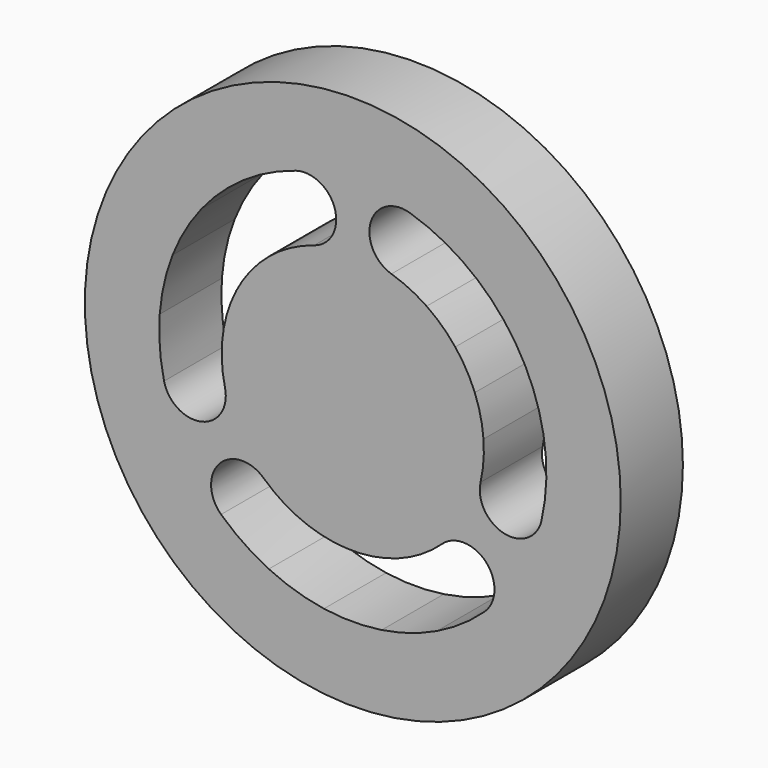
from build123d import *

# Parameters (mm, degrees)
F0_R     = 38.1
F1_DEPTH = 11.049
F3_DEPTH = 11.05


with BuildPart() as f1:
    # F0 (on Front) → F1 (new body)
    with BuildSketch(Plane.XZ):
        Circle(F0_R)
    extrude(amount=F1_DEPTH)

    # F2 (on face) → F3 (cut, through all)
    with BuildSketch(Plane.XZ.offset(11.049)):
        with BuildLine():
            ThreePointArc((-5.4934258743, 17.8092492746), (-3.2271754935, 19.4172396715), (-2.3586126245, 22.0567703964))
            ThreePointArc((-2.3586126245, 22.0567703964), (-4.1640818997, 25.6332075274), (-8.1137993748, 26.3042915181))
            ThreePointArc((-8.1137993748, 26.3042915181), (-10.0430162679, 25.1004998579), (-11.1244292478, 23.1001153577))
            ThreePointArc((-11.1244292478, 23.1001153577), (-9.253900361, 21.4598737334), (-8.5576944102, 19.0714499485))
            ThreePointArc((-8.5576944102, 19.0714499485), (-8.5888494373, 18.5460952541), (-8.681877787, 18.0281049871))
            ThreePointArc((-8.681877787, 18.0281049871), (-7.108001728, 17.6222047723), (-5.4934258743, 17.8092492746))
        make_face()
        with BuildLine():
            ThreePointArc((-11.1244292478, 23.1001153577), (-10.0430162679, 25.1004998579), (-8.1137993748, 26.3042915181))
            ThreePointArc((-8.1137993748, 26.3042915181), (-11.9436262917, 24.8011952044), (-15.5066523142, 22.7440811326))
            ThreePointArc((-15.5066523142, 22.7440811326), (-13.36264294, 23.5018519681), (-11.1244292478, 23.1001153577))
        make_face()
        with BuildLine():
            ThreePointArc((-10.498736832, 15.3988185422), (-8.0863997604, 16.7915820124), (-5.4934258743, 17.8092492746))
            ThreePointArc((-5.4934258743, 17.8092492746), (-7.108001728, 17.6222047723), (-8.681877787, 18.0281049871))
            ThreePointArc((-8.681877787, 18.0281049871), (-9.34582792, 16.5445244505), (-10.498736832, 15.3988185422))
        make_face()
        with BuildLine():
            ThreePointArc((-8.5576944102, 19.0714499485), (-9.253900361, 21.4598737334), (-11.1244292478, 23.1001153577))
            ThreePointArc((-11.1244292478, 23.1001153577), (-10.8084192424, 20.128157176), (-8.681877787, 18.0281049871))
            ThreePointArc((-8.681877787, 18.0281049871), (-8.5888494373, 18.5460952541), (-8.5576944102, 19.0714499485))
        make_face()
        with BuildLine():
            ThreePointArc((-8.681877787, 18.0281049871), (-10.8084192424, 20.128157176), (-11.1244292478, 23.1001153577))
            ThreePointArc((-11.1244292478, 23.1001153577), (-13.36264294, 23.5018519681), (-15.5066523142, 22.7440811326))
            ThreePointArc((-15.5066523142, 22.7440811326), (-16.9953355125, 21.0251239305), (-17.4390806002, 18.7948589632))
            ThreePointArc((-17.4390806002, 18.7948589632), (-14.7880141659, 17.4149152983), (-13.6100435462, 14.6681384642))
            ThreePointArc((-13.6100435462, 14.6681384642), (-11.986449243, 14.7441793583), (-10.498736832, 15.3988185422))
            ThreePointArc((-10.498736832, 15.3988185422), (-9.34582792, 16.5445244505), (-8.681877787, 18.0281049871))
        make_face()
        with BuildLine():
            ThreePointArc((-17.4390806002, 18.7948589632), (-16.9953355125, 21.0251239305), (-15.5066523142, 22.7440811326))
            ThreePointArc((-15.5066523142, 22.7440811326), (-18.7232851045, 20.178902038), (-21.5216706751, 17.1629596491))
            ThreePointArc((-21.5216706751, 17.1629596491), (-19.696270544, 18.5190225314), (-17.4390806002, 18.7948589632))
        make_face()
        with BuildLine():
            ThreePointArc((-14.571188844, 11.6201352503), (-12.6765494203, 13.6620709396), (-10.498736832, 15.3988185422))
            ThreePointArc((-10.498736832, 15.3988185422), (-11.986449243, 14.7441793583), (-13.6100435462, 14.6681384642))
            ThreePointArc((-13.6100435462, 14.6681384642), (-13.6035837106, 14.5299100198), (-13.6014297362, 14.391547479))
            ThreePointArc((-13.6014297362, 14.391547479), (-13.8508683455, 12.9234570127), (-14.571188844, 11.6201352503))
        make_face()
        with BuildLine():
            ThreePointArc((-13.6100435462, 14.6681384642), (-14.7880141659, 17.4149152983), (-17.4390806002, 18.7948589632))
            ThreePointArc((-17.4390806002, 18.7948589632), (-16.2611099805, 16.0480821291), (-13.6100435462, 14.6681384642))
        make_face()
        with BuildLine():
            ThreePointArc((-13.6100435462, 14.6681384642), (-16.2611099805, 16.0480821291), (-17.4390806002, 18.7948589632))
            ThreePointArc((-17.4390806002, 18.7948589632), (-19.696270544, 18.5190225314), (-21.5216706751, 17.1629596491))
            ThreePointArc((-21.5216706751, 17.1629596491), (-22.437544489, 15.0815737307), (-22.2041931112, 12.8195968699))
            ThreePointArc((-22.2041931112, 12.8195968699), (-19.2641605846, 12.2823757795), (-17.3288972096, 10.0048434687))
            ThreePointArc((-17.3288972096, 10.0048434687), (-15.7998480839, 10.5560689065), (-14.571188844, 11.6201352503))
            ThreePointArc((-14.571188844, 11.6201352503), (-13.8508683455, 12.9234570127), (-13.6014297362, 14.391547479))
            ThreePointArc((-13.6014297362, 14.391547479), (-13.6035837106, 14.5299100198), (-13.6100435462, 14.6681384642))
        make_face()
        with BuildLine():
            ThreePointArc((-22.2041931112, 12.8195968699), (-22.437544489, 15.0815737307), (-21.5216706751, 17.1629596491))
            ThreePointArc((-21.5216706751, 17.1629596491), (-23.8392977721, 13.7636250419), (-25.6243943624, 10.0568338021))
            ThreePointArc((-25.6243943624, 10.0568338021), (-24.2797981866, 11.8906966911), (-22.2041931112, 12.8195968699))
        make_face()
        with BuildLine():
            ThreePointArc((-17.3489268741, 6.8089517461), (-16.1403320456, 9.3186248461), (-14.571188844, 11.6201352503))
            ThreePointArc((-14.571188844, 11.6201352503), (-15.7998480839, 10.5560689065), (-17.3288972096, 10.0048434687))
            ThreePointArc((-17.3288972096, 10.0048434687), (-17.114059345, 9.2318818452), (-17.0416605846, 8.4328928597))
            ThreePointArc((-17.0416605846, 8.4328928597), (-17.1191526371, 7.6065156285), (-17.3489268741, 6.8089517461))
        make_face()
        with BuildLine():
            ThreePointArc((-17.3288972096, 10.0048434687), (-19.2641605846, 12.2823757795), (-22.2041931112, 12.8195968699))
            ThreePointArc((-22.2041931112, 12.8195968699), (-20.2689297362, 10.5420645591), (-17.3288972096, 10.0048434687))
        make_face()
        with BuildLine():
            ThreePointArc((-17.3288972096, 10.0048434687), (-20.2689297362, 10.5420645591), (-22.2041931112, 12.8195968699))
            ThreePointArc((-22.2041931112, 12.8195968699), (-24.2797981866, 11.8906966911), (-25.6243943624, 10.0568338021))
            ThreePointArc((-25.6243943624, 10.0568338021), (-25.8860792444, 7.7979594331), (-24.9963656228, 5.7052573369))
            ThreePointArc((-24.9963656228, 5.7052573369), (-22.028601796, 6.0584932723), (-19.5080023094, 4.4525742255))
            ThreePointArc((-19.5080023094, 4.4525742255), (-18.209361165, 5.4300053303), (-17.3489268741, 6.8089517461))
            ThreePointArc((-17.3489268741, 6.8089517461), (-17.1191526371, 7.6065156285), (-17.0416605846, 8.4328928597))
            ThreePointArc((-17.0416605846, 8.4328928597), (-17.114059345, 9.2318818452), (-17.3288972096, 10.0048434687))
        make_face()
        with BuildLine():
            ThreePointArc((-24.9963656228, 5.7052573369), (-25.8860792444, 7.7979594331), (-25.6243943624, 10.0568338021))
            ThreePointArc((-25.6243943624, 10.0568338021), (-26.8370843559, 6.1253894436), (-27.4502782232, 2.0571140049))
            ThreePointArc((-27.4502782232, 2.0571140049), (-26.7059592707, 4.205830226), (-24.9963656228, 5.7052573369))
        make_face()
        with BuildLine():
            ThreePointArc((-18.5851364875, 1.3927631904), (-18.1699752899, 4.1471780197), (-17.3489268741, 6.8089517461))
            ThreePointArc((-17.3489268741, 6.8089517461), (-18.209361165, 5.4300053303), (-19.5080023094, 4.4525742255))
            ThreePointArc((-19.5080023094, 4.4525742255), (-18.81302758, 3.1667060392), (-18.5727073475, 1.7249387027))
            ThreePointArc((-18.5727073475, 1.7249387027), (-18.5758157193, 1.5587347207), (-18.5851364875, 1.3927631904))
        make_face()
        with BuildLine():
            ThreePointArc((-19.5080023094, 4.4525742255), (-22.028601796, 6.0584932723), (-24.9963656228, 5.7052573369))
            ThreePointArc((-24.9963656228, 5.7052573369), (-22.4757661361, 4.09933829), (-19.5080023094, 4.4525742255))
        make_face()
        with BuildLine():
            ThreePointArc((-19.5080023094, 4.4525742255), (-22.4757661361, 4.09933829), (-24.9963656228, 5.7052573369))
            ThreePointArc((-24.9963656228, 5.7052573369), (-26.7059592707, 4.205830226), (-27.4502782232, 2.0571140049))
            ThreePointArc((-27.4502782232, 2.0571140049), (-27.0345222544, -0.1785378544), (-25.567501354, -1.9160193477))
            ThreePointArc((-25.567501354, -1.9160193477), (-22.835705067, -0.7037129493), (-19.9537357944, -1.4953257775))
            ThreePointArc((-19.9537357944, -1.4953257775), (-19.0008925012, -0.1785379824), (-18.5851364875, 1.3927631904))
            ThreePointArc((-18.5851364875, 1.3927631904), (-18.5758157193, 1.5587347207), (-18.5727073475, 1.7249387027))
            ThreePointArc((-18.5727073475, 1.7249387027), (-18.81302758, 3.1667060392), (-19.5080023094, 4.4525742255))
        make_face()
        with BuildLine():
            ThreePointArc((-25.567501354, -1.9160193477), (-27.0345222544, -0.1785378544), (-27.4502782232, 2.0571140049))
            ThreePointArc((-27.4502782232, 2.0571140049), (-27.4502782273, -2.0571139506), (-26.8370843706, -6.1253893792))
            ThreePointArc((-26.8370843706, -6.1253893792), (-26.7591786586, -3.8527427103), (-25.567501354, -1.9160193477))
        make_face()
        with BuildLine():
            ThreePointArc((-18.1699752313, -4.1471782764), (-18.5851364598, -1.3927635598), (-18.5851364875, 1.3927631904))
            ThreePointArc((-18.5851364875, 1.3927631904), (-19.0008925012, -0.1785379824), (-19.9537357944, -1.4953257775))
            ThreePointArc((-19.9537357944, -1.4953257775), (-18.8152778676, -2.6553923195), (-18.1699752313, -4.1471782764))
        make_face()
        with BuildLine():
            ThreePointArc((-19.9537357944, -1.4953257775), (-22.835705067, -0.7037129493), (-25.567501354, -1.9160193477))
            ThreePointArc((-25.567501354, -1.9160193477), (-22.6855320815, -2.7076321758), (-19.9537357944, -1.4953257775))
        make_face()
        with BuildLine():
            ThreePointArc((-19.9537357944, -1.4953257775), (-22.6855320815, -2.7076321758), (-25.567501354, -1.9160193477))
            ThreePointArc((-25.567501354, -1.9160193477), (-26.7591786586, -3.8527427103), (-26.8370843706, -6.1253893792))
            ThreePointArc((-26.8370843706, -6.1253893792), (-22.0058477047, -9.5533346008), (-18.058529801, -5.1362838278))
            ThreePointArc((-18.058529801, -5.1362838278), (-18.086479028, -4.6386017315), (-18.1699752313, -4.1471782764))
            ThreePointArc((-18.1699752313, -4.1471782764), (-18.8152778676, -2.6553923195), (-19.9537357944, -1.4953257775))
        make_face()
        with BuildLine():
            ThreePointArc((-11.2718580074, -16.5327792097), (-11.7072761395, -14.9668124528), (-12.676549357, -13.6620709983))
            ThreePointArc((-12.676549357, -13.6620709983), (-18.9583327467, -13.8971187492), (-18.7232849958, -20.1789021388))
            ThreePointArc((-18.7232849958, -20.1789021388), (-16.7161623907, -21.2477571476), (-14.4430721062, -21.18409601))
            ThreePointArc((-14.4430721062, -21.18409601), (-13.6876442891, -18.292430993), (-11.2718580074, -16.5327792097))
        make_face()
        with BuildLine():
            ThreePointArc((-8.0863997947, -16.7915819959), (-10.4987367878, -15.3988185723), (-12.676549357, -13.6620709983))
            ThreePointArc((-12.676549357, -13.6620709983), (-11.7072761395, -14.9668124528), (-11.2718580074, -16.5327792097))
            ThreePointArc((-11.2718580074, -16.5327792097), (-9.6550645989, -16.3659866159), (-8.0863997947, -16.7915819959))
        make_face()
        with BuildLine():
            ThreePointArc((-14.4430721062, -21.18409601), (-16.7161623907, -21.2477571476), (-18.7232849958, -20.1789021388))
            ThreePointArc((-18.7232849958, -20.1789021388), (-15.5066520681, -22.7440813004), (-11.9436261572, -24.8011952692))
            ThreePointArc((-11.9436261572, -24.8011952692), (-13.6718794549, -23.3233141096), (-14.4430721062, -21.18409601))
        make_face()
        with BuildLine():
            ThreePointArc((-8.0863997947, -16.7915819959), (-9.6550645989, -16.3659866159), (-11.2718580074, -16.5327792097))
            ThreePointArc((-11.2718580074, -16.5327792097), (-11.2591544038, -16.7264479204), (-11.2549171764, -16.9204865685))
            ThreePointArc((-11.2549171764, -16.9204865685), (-12.1400926486, -19.5823795663), (-14.4430721062, -21.18409601))
            ThreePointArc((-14.4430721062, -21.18409601), (-13.6718794549, -23.3233141096), (-11.9436261572, -24.8011952692))
            ThreePointArc((-11.9436261572, -24.8011952692), (-9.7106238335, -25.2309542751), (-7.5572850225, -24.5001163))
            ThreePointArc((-7.5572850225, -24.5001163), (-7.6877519702, -21.5142535884), (-5.8979587632, -19.1207126897))
            ThreePointArc((-5.8979587632, -19.1207126897), (-6.7756093234, -17.7526591581), (-8.0863997947, -16.7915819959))
        make_face()
        with BuildLine():
            ThreePointArc((-11.2549171764, -16.9204865685), (-11.2591544038, -16.7264479204), (-11.2718580074, -16.5327792097))
            ThreePointArc((-11.2718580074, -16.5327792097), (-13.6876442891, -18.292430993), (-14.4430721062, -21.18409601))
            ThreePointArc((-14.4430721062, -21.18409601), (-12.1400926486, -19.5823795663), (-11.2549171764, -16.9204865685))
        make_face()
        with BuildLine():
            ThreePointArc((-2.777738202, -18.4290872819), (-5.4934260251, -17.8092492281), (-8.0863997947, -16.7915819959))
            ThreePointArc((-8.0863997947, -16.7915819959), (-6.7756093234, -17.7526591581), (-5.8979587632, -19.1207126897))
            ThreePointArc((-5.8979587632, -19.1207126897), (-4.4021579991, -18.4847720153), (-2.777738202, -18.4290872819))
        make_face()
        with BuildLine():
            ThreePointArc((-7.5572850225, -24.5001163), (-9.7106238335, -25.2309542751), (-11.9436261572, -24.8011952692))
            ThreePointArc((-11.9436261572, -24.8011952692), (-8.1137993206, -26.3042915348), (-4.10272361, -27.219793378))
            ThreePointArc((-4.10272361, -27.219793378), (-6.1898086487, -26.3169819519), (-7.5572850225, -24.5001163))
        make_face()
        with BuildLine():
            ThreePointArc((-2.777738202, -18.4290872819), (-4.4021579991, -18.4847720153), (-5.8979587632, -19.1207126897))
            ThreePointArc((-5.8979587632, -19.1207126897), (-5.6527697755, -19.9426559072), (-5.5700129372, -20.7963886511))
            ThreePointArc((-5.5700129372, -20.7963886511), (-6.0982141435, -22.8979861886), (-7.5572850225, -24.5001163))
            ThreePointArc((-7.5572850225, -24.5001163), (-6.1898086487, -26.3169819519), (-4.10272361, -27.219793378))
            ThreePointArc((-4.10272361, -27.219793378), (-1.8422536822, -26.9722703708), (0, -25.6391937398))
            ThreePointArc((0, -25.6391937398), (-1.0047691516, -22.8244403386), (0, -20.0096869375))
            ThreePointArc((0, -20.0096869375), (-1.2418999278, -18.9611041944), (-2.777738202, -18.4290872819))
        make_face()
        with BuildLine():
            ThreePointArc((-5.5700129372, -20.7963886511), (-5.6527697755, -19.9426559072), (-5.8979587632, -19.1207126897))
            ThreePointArc((-5.8979587632, -19.1207126897), (-7.6877519702, -21.5142535884), (-7.5572850225, -24.5001163))
            ThreePointArc((-7.5572850225, -24.5001163), (-6.0982141435, -22.8979861886), (-5.5700129372, -20.7963886511))
        make_face()
        with BuildLine():
            ThreePointArc((2.7777382002, -18.4290872822), (-9e-10, -18.63725), (-2.777738202, -18.4290872819))
            ThreePointArc((-2.777738202, -18.4290872819), (-1.2418999278, -18.9611041944), (0, -20.0096869375))
            ThreePointArc((0, -20.0096869375), (1.241899927, -18.9611041949), (2.7777382002, -18.4290872822))
        make_face()
        with BuildLine():
            ThreePointArc((0, -25.6391937398), (-1.8422536822, -26.9722703708), (-4.10272361, -27.219793378))
            ThreePointArc((-4.10272361, -27.219793378), (3e-10, -27.52725), (4.1027236105, -27.219793378))
            ThreePointArc((4.1027236105, -27.219793378), (1.8422536824, -26.9722703709), (0, -25.6391937398))
        make_face()
        with BuildLine():
            ThreePointArc((2.7777382002, -18.4290872822), (1.241899927, -18.9611041949), (0, -20.0096869375))
            ThreePointArc((0, -20.0096869375), (0.7460473985, -21.3300844776), (1.0047691516, -22.8244403386))
            ThreePointArc((1.0047691516, -22.8244403386), (0.7460473985, -24.3187961996), (0, -25.6391937398))
            ThreePointArc((0, -25.6391937398), (1.8422536824, -26.9722703709), (4.1027236105, -27.219793378))
            ThreePointArc((4.1027236105, -27.219793378), (6.1898086489, -26.3169819518), (7.5572850225, -24.5001163))
            ThreePointArc((7.5572850225, -24.5001163), (5.7674918155, -22.1065754014), (5.8979587632, -19.1207126897))
            ThreePointArc((5.8979587632, -19.1207126897), (4.4021579983, -18.4847720151), (2.7777382002, -18.4290872822))
        make_face()
        with BuildLine():
            ThreePointArc((1.0047691516, -22.8244403386), (0.7460473985, -21.3300844776), (0, -20.0096869375))
            ThreePointArc((0, -20.0096869375), (-1.0047691516, -22.8244403386), (0, -25.6391937398))
            ThreePointArc((0, -25.6391937398), (0.7460473985, -24.3187961996), (1.0047691516, -22.8244403386))
        make_face()
        with BuildLine():
            ThreePointArc((8.0863994561, -16.7915821589), (5.4934258447, -17.8092492838), (2.7777382002, -18.4290872822))
            ThreePointArc((2.7777382002, -18.4290872822), (4.4021579983, -18.4847720151), (5.8979587632, -19.1207126897))
            ThreePointArc((5.8979587632, -19.1207126897), (6.7756091948, -17.752659295), (8.0863994561, -16.7915821589))
        make_face()
        with BuildLine():
            ThreePointArc((7.5572850225, -24.5001163), (6.1898086489, -26.3169819518), (4.1027236105, -27.219793378))
            ThreePointArc((4.1027236105, -27.219793378), (8.1137992679, -26.3042915511), (11.9436260573, -24.8011953173))
            ThreePointArc((11.9436260573, -24.8011953173), (9.7106237782, -25.2309542713), (7.5572850225, -24.5001163))
        make_face()
        with BuildLine():
            ThreePointArc((8.0863994561, -16.7915821589), (6.7756091948, -17.752659295), (5.8979587632, -19.1207126897))
            ThreePointArc((5.8979587632, -19.1207126897), (7.3570296422, -20.7228428012), (7.8852308484, -22.8244403386))
            ThreePointArc((7.8852308484, -22.8244403386), (7.8024740102, -23.6781730826), (7.5572850225, -24.5001163))
            ThreePointArc((7.5572850225, -24.5001163), (9.7106237782, -25.2309542713), (11.9436260573, -24.8011953173))
            ThreePointArc((11.9436260573, -24.8011953173), (13.6718794233, -23.3233141552), (14.4430721062, -21.18409601))
            ThreePointArc((14.4430721062, -21.18409601), (12.0272858246, -19.4244442266), (11.2718580074, -16.5327792097))
            ThreePointArc((11.2718580074, -16.5327792097), (9.6550644116, -16.3659866311), (8.0863994561, -16.7915821589))
        make_face()
        with BuildLine():
            ThreePointArc((7.8852308484, -22.8244403386), (7.3570296422, -20.7228428012), (5.8979587632, -19.1207126897))
            ThreePointArc((5.8979587632, -19.1207126897), (5.7674918155, -22.1065754014), (7.5572850225, -24.5001163))
            ThreePointArc((7.5572850225, -24.5001163), (7.8024740102, -23.6781730826), (7.8852308484, -22.8244403386))
        make_face()
        with BuildLine():
            ThreePointArc((12.676549357, -13.6620709983), (10.4987366326, -15.3988186781), (8.0863994561, -16.7915821589))
            ThreePointArc((8.0863994561, -16.7915821589), (9.6550644116, -16.3659866311), (11.2718580074, -16.5327792097))
            ThreePointArc((11.2718580074, -16.5327792097), (11.7072761395, -14.9668124528), (12.676549357, -13.6620709983))
        make_face()
        with BuildLine():
            ThreePointArc((14.4430721062, -21.18409601), (13.6718794233, -23.3233141552), (11.9436260573, -24.8011953173))
            ThreePointArc((11.9436260573, -24.8011953173), (15.5066520223, -22.7440813317), (18.7232849958, -20.1789021388))
            ThreePointArc((18.7232849958, -20.1789021388), (16.7161623907, -21.2477571476), (14.4430721062, -21.18409601))
        make_face()
        with BuildLine():
            ThreePointArc((12.676549357, -13.6620709983), (11.7072761395, -14.9668124528), (11.2718580074, -16.5327792097))
            ThreePointArc((11.2718580074, -16.5327792097), (13.574837465, -18.1344956534), (14.4600129372, -20.7963886511))
            ThreePointArc((14.4600129372, -20.7963886511), (14.4557757099, -20.9904272993), (14.4430721062, -21.18409601))
            ThreePointArc((14.4430721062, -21.18409601), (16.7161623907, -21.2477571476), (18.7232849958, -20.1789021388))
            ThreePointArc((18.7232849958, -20.1789021388), (19.7740364038, -18.6980066166), (20.1449171764, -16.9204865685))
            ThreePointArc((20.1449171764, -16.9204865685), (17.4774372245, -12.8463673412), (12.676549357, -13.6620709983))
        make_face()
        with BuildLine():
            ThreePointArc((14.4600129372, -20.7963886511), (13.574837465, -18.1344956534), (11.2718580074, -16.5327792097))
            ThreePointArc((11.2718580074, -16.5327792097), (12.0272858246, -19.4244442266), (14.4430721062, -21.18409601))
            ThreePointArc((14.4430721062, -21.18409601), (14.4557757099, -20.9904272993), (14.4600129372, -20.7963886511))
        make_face()
        with BuildLine():
            ThreePointArc((19.9537357944, -1.4953257775), (18.8152778676, -2.6553923195), (18.1699752313, -4.1471782764))
            ThreePointArc((18.1699752313, -4.1471782764), (21.5144242495, -9.4698383975), (26.8370843706, -6.1253893792))
            ThreePointArc((26.8370843706, -6.1253893792), (26.9205805739, -5.6339659241), (26.948529801, -5.1362838278))
            ThreePointArc((26.948529801, -5.1362838278), (26.5887090231, -3.3843318526), (25.567501354, -1.9160193477))
            ThreePointArc((25.567501354, -1.9160193477), (22.6855320815, -2.7076321758), (19.9537357944, -1.4953257775))
        make_face()
        with BuildLine():
            ThreePointArc((18.5851364872, 1.3927631935), (18.5851364599, -1.3927635583), (18.1699752313, -4.1471782764))
            ThreePointArc((18.1699752313, -4.1471782764), (18.8152778676, -2.6553923195), (19.9537357944, -1.4953257775))
            ThreePointArc((19.9537357944, -1.4953257775), (19.0008925005, -0.178537981), (18.5851364872, 1.3927631935))
        make_face()
        with BuildLine():
            ThreePointArc((26.948529801, -5.1362838278), (26.9205805739, -5.6339659241), (26.8370843706, -6.1253893792))
            ThreePointArc((26.8370843706, -6.1253893792), (27.4502782184, -2.0571140698), (27.4502782411, 2.0571137665))
            ThreePointArc((27.4502782411, 2.0571137665), (27.4595989841, 1.8911424599), (27.4627073475, 1.7249387027))
            ThreePointArc((27.4627073475, 1.7249387027), (26.9605400449, -0.327400285), (25.567501354, -1.9160193477))
            ThreePointArc((25.567501354, -1.9160193477), (26.5887090231, -3.3843318526), (26.948529801, -5.1362838278))
        make_face()
        with BuildLine():
            ThreePointArc((18.5851364872, 1.3927631935), (19.0008925005, -0.178537981), (19.9537357944, -1.4953257775))
            ThreePointArc((19.9537357944, -1.4953257775), (22.835705067, -0.7037129493), (25.567501354, -1.9160193477))
            ThreePointArc((25.567501354, -1.9160193477), (26.9605400449, -0.327400285), (27.4627073475, 1.7249387027))
            ThreePointArc((27.4627073475, 1.7249387027), (27.4595989841, 1.8911424599), (27.4502782411, 2.0571137665))
            ThreePointArc((27.4502782411, 2.0571137665), (26.7059593375, 4.2058301268), (24.9963656228, 5.7052573369))
            ThreePointArc((24.9963656228, 5.7052573369), (22.4757661361, 4.09933829), (19.5080023094, 4.4525742255))
            ThreePointArc((19.5080023094, 4.4525742255), (18.7620584546, 3.0084797035), (18.5851364872, 1.3927631935))
        make_face()
        with BuildLine():
            ThreePointArc((25.567501354, -1.9160193477), (22.835705067, -0.7037129493), (19.9537357944, -1.4953257775))
            ThreePointArc((19.9537357944, -1.4953257775), (22.6855320815, -2.7076321758), (25.567501354, -1.9160193477))
        make_face()
        with BuildLine():
            ThreePointArc((17.3489268739, 6.8089517465), (18.1699752895, 4.1471780214), (18.5851364872, 1.3927631935))
            ThreePointArc((18.5851364872, 1.3927631935), (18.7620584546, 3.0084797035), (19.5080023094, 4.4525742255))
            ThreePointArc((19.5080023094, 4.4525742255), (18.2093611648, 5.4300053305), (17.3489268739, 6.8089517465))
        make_face()
        with BuildLine():
            ThreePointArc((24.9963656228, 5.7052573369), (26.7059593375, 4.2058301268), (27.4502782411, 2.0571137665))
            ThreePointArc((27.4502782411, 2.0571137665), (26.8370843933, 6.12538928), (25.6243943976, 10.0568337123))
            ThreePointArc((25.6243943976, 10.0568337123), (25.8541685582, 9.2592699531), (25.9316605846, 8.4328928597))
            ThreePointArc((25.9316605846, 8.4328928597), (25.6913403521, 6.9911255231), (24.9963656228, 5.7052573369))
        make_face()
        with BuildLine():
            ThreePointArc((17.3489268739, 6.8089517465), (18.2093611648, 5.4300053305), (19.5080023094, 4.4525742255))
            ThreePointArc((19.5080023094, 4.4525742255), (22.028601796, 6.0584932723), (24.9963656228, 5.7052573369))
            ThreePointArc((24.9963656228, 5.7052573369), (25.6913403521, 6.9911255231), (25.9316605846, 8.4328928597))
            ThreePointArc((25.9316605846, 8.4328928597), (25.8541685582, 9.2592699531), (25.6243943976, 10.0568337123))
            ThreePointArc((25.6243943976, 10.0568337123), (24.2797982242, 11.8906966607), (22.2041931112, 12.8195968699))
            ThreePointArc((22.2041931112, 12.8195968699), (20.2689297362, 10.5420645591), (17.3288972096, 10.0048434687))
            ThreePointArc((17.3288972096, 10.0048434687), (17.0417478802, 8.4050351858), (17.3489268739, 6.8089517465))
        make_face()
        with BuildLine():
            ThreePointArc((24.9963656228, 5.7052573369), (22.028601796, 6.0584932723), (19.5080023094, 4.4525742255))
            ThreePointArc((19.5080023094, 4.4525742255), (22.4757661361, 4.09933829), (24.9963656228, 5.7052573369))
        make_face()
        with BuildLine():
            ThreePointArc((14.5711889608, 11.6201351039), (16.1403320923, 9.3186247651), (17.3489268739, 6.8089517465))
            ThreePointArc((17.3489268739, 6.8089517465), (17.0417478802, 8.4050351858), (17.3288972096, 10.0048434687))
            ThreePointArc((17.3288972096, 10.0048434687), (15.7998481648, 10.5560688592), (14.5711889608, 11.6201351039))
        make_face()
        with BuildLine():
            ThreePointArc((22.2041931112, 12.8195968699), (24.2797982242, 11.8906966607), (25.6243943976, 10.0568337123))
            ThreePointArc((25.6243943976, 10.0568337123), (23.8392978471, 13.763624912), (21.521670802, 17.1629594899))
            ThreePointArc((21.521670802, 17.1629594899), (22.2419911729, 15.8596378138), (22.4914297362, 14.391547479))
            ThreePointArc((22.4914297362, 14.391547479), (22.4190309758, 13.5925584934), (22.2041931112, 12.8195968699))
        make_face()
        with BuildLine():
            ThreePointArc((14.5711889608, 11.6201351039), (15.7998481648, 10.5560688592), (17.3288972096, 10.0048434687))
            ThreePointArc((17.3288972096, 10.0048434687), (19.2641605846, 12.2823757795), (22.2041931112, 12.8195968699))
            ThreePointArc((22.2041931112, 12.8195968699), (22.4190309758, 13.5925584934), (22.4914297362, 14.391547479))
            ThreePointArc((22.4914297362, 14.391547479), (22.2419911729, 15.8596378138), (21.521670802, 17.1629594899))
            ThreePointArc((21.521670802, 17.1629594899), (19.6962706385, 18.5190224936), (17.4390806002, 18.7948589632))
            ThreePointArc((17.4390806002, 18.7948589632), (16.2611099805, 16.0480821291), (13.6100435462, 14.6681384642))
            ThreePointArc((13.6100435462, 14.6681384642), (13.8072032229, 13.0547664315), (14.5711889608, 11.6201351039))
        make_face()
        with BuildLine():
            ThreePointArc((22.2041931112, 12.8195968699), (19.2641605846, 12.2823757795), (17.3288972096, 10.0048434687))
            ThreePointArc((17.3288972096, 10.0048434687), (20.2689297362, 10.5420645591), (22.2041931112, 12.8195968699))
        make_face()
        with BuildLine():
            ThreePointArc((10.4987366772, 15.3988186477), (12.6765494203, 13.6620709396), (14.5711889608, 11.6201351039))
            ThreePointArc((14.5711889608, 11.6201351039), (13.8072032229, 13.0547664315), (13.6100435462, 14.6681384642))
            ThreePointArc((13.6100435462, 14.6681384642), (11.9864491518, 14.7441793798), (10.4987366772, 15.3988186477))
        make_face()
        with BuildLine():
            ThreePointArc((17.4390806002, 18.7948589632), (19.6962706385, 18.5190224936), (21.521670802, 17.1629594899))
            ThreePointArc((21.521670802, 17.1629594899), (18.7232849234, 20.1789022061), (15.5066517377, 22.7440815257))
            ThreePointArc((15.5066517377, 22.7440815257), (16.9325872409, 21.148459178), (17.4476944102, 19.0714499485))
            ThreePointArc((17.4476944102, 19.0714499485), (17.4455404358, 18.9330874076), (17.4390806002, 18.7948589632))
        make_face()
        with BuildLine():
            ThreePointArc((10.4987366772, 15.3988186477), (11.9864491518, 14.7441793798), (13.6100435462, 14.6681384642))
            ThreePointArc((13.6100435462, 14.6681384642), (14.7880141659, 17.4149152983), (17.4390806002, 18.7948589632))
            ThreePointArc((17.4390806002, 18.7948589632), (17.4455404358, 18.9330874076), (17.4476944102, 19.0714499485))
            ThreePointArc((17.4476944102, 19.0714499485), (16.9325872409, 21.148459178), (15.5066517377, 22.7440815257))
            ThreePointArc((15.5066517377, 22.7440815257), (13.3626425922, 23.5018519964), (11.1244292478, 23.1001153577))
            ThreePointArc((11.1244292478, 23.1001153577), (11.2174575975, 22.5821250907), (11.2486126245, 22.0567703964))
            ThreePointArc((11.2486126245, 22.0567703964), (10.5524066738, 19.6683466114), (8.681877787, 18.0281049871))
            ThreePointArc((8.681877787, 18.0281049871), (9.3458278667, 16.5445245275), (10.4987366772, 15.3988186477))
        make_face()
        with BuildLine():
            ThreePointArc((17.4390806002, 18.7948589632), (14.7880141659, 17.4149152983), (13.6100435462, 14.6681384642))
            ThreePointArc((13.6100435462, 14.6681384642), (16.2611099805, 16.0480821291), (17.4390806002, 18.7948589632))
        make_face()
        with BuildLine():
            ThreePointArc((5.4934258743, 17.8092492746), (8.086399676, 16.791582053), (10.4987366772, 15.3988186477))
            ThreePointArc((10.4987366772, 15.3988186477), (9.3458278667, 16.5445245275), (8.681877787, 18.0281049871))
            ThreePointArc((8.681877787, 18.0281049871), (7.108001728, 17.6222047723), (5.4934258743, 17.8092492746))
        make_face()
        with BuildLine():
            ThreePointArc((11.1244292478, 23.1001153577), (13.3626425922, 23.5018519964), (15.5066517377, 22.7440815257))
            ThreePointArc((15.5066517377, 22.7440815257), (11.9436259774, 24.8011953558), (8.1137993748, 26.3042915181))
            ThreePointArc((8.1137993748, 26.3042915181), (10.0430162679, 25.1004998579), (11.1244292478, 23.1001153577))
        make_face()
        with BuildLine():
            ThreePointArc((5.4934258743, 17.8092492746), (7.108001728, 17.6222047723), (8.681877787, 18.0281049871))
            ThreePointArc((8.681877787, 18.0281049871), (8.9978877924, 21.0000631688), (11.1244292478, 23.1001153577))
            ThreePointArc((11.1244292478, 23.1001153577), (10.0430162679, 25.1004998579), (8.1137993748, 26.3042915181))
            ThreePointArc((8.1137993748, 26.3042915181), (2.5560915028, 23.3669571466), (5.4934258743, 17.8092492746))
        make_face()
        with BuildLine():
            ThreePointArc((11.1244292478, 23.1001153577), (8.9978877924, 21.0000631688), (8.681877787, 18.0281049871))
            ThreePointArc((8.681877787, 18.0281049871), (10.5524066738, 19.6683466114), (11.2486126245, 22.0567703964))
            ThreePointArc((11.2486126245, 22.0567703964), (11.2174575975, 22.5821250907), (11.1244292478, 23.1001153577))
        make_face()
    extrude(amount=-F3_DEPTH, mode=Mode.SUBTRACT)


solid = f1.part
